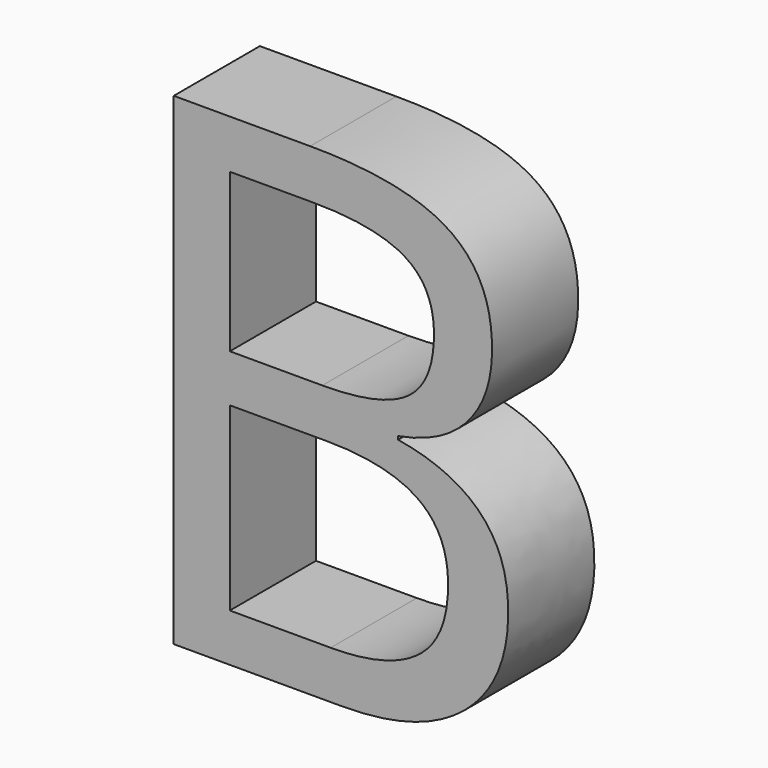
from build123d import *

# Parameters (mm, degrees)
F0_TEXT_SIZE = 159.5070947789
F1_DEPTH     = 25.4


# Not quite as in the source:
# - Text() gives the source's letters only with a copy of the font that has no kerning and outlines rounded to 1/6400 em; it was checked with that copy


with BuildPart() as f1:
    # F0 (on Front) → F1 (new body)
    with BuildSketch(Plane.XZ):
        with Locations((-47.4286675453, -57.5919449329)):
            Text('B', F0_TEXT_SIZE, font='Open Sans', text_align=(TextAlign.LEFT, TextAlign.BOTTOM))
    extrude(amount=F1_DEPTH)


solid = f1.part
